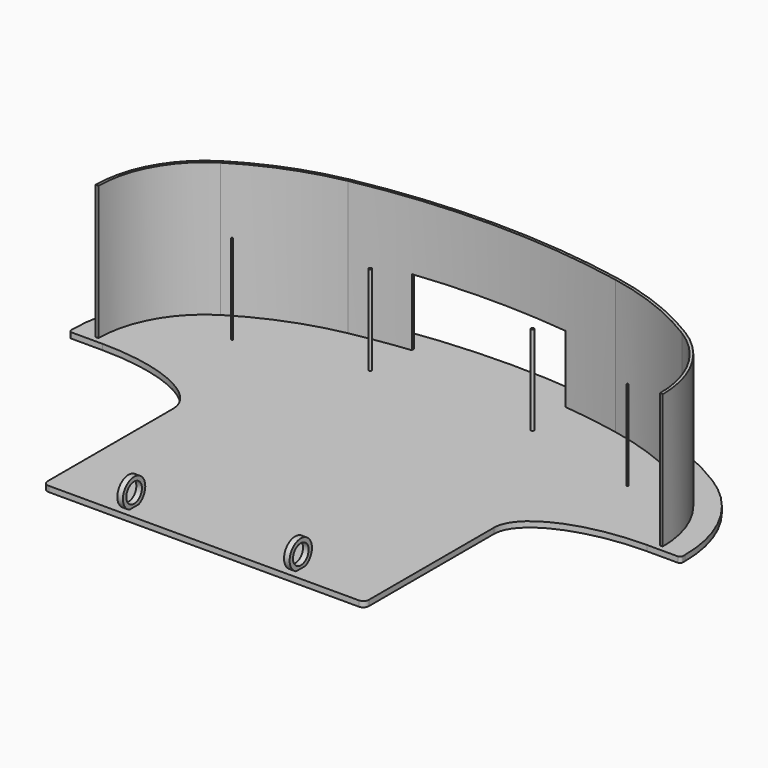
from build123d import *

# Parameters (mm, degrees)
F1_DEPTH  = 12.7
F3_R      = 31.75
F3_R_2    = 22.225
F4_DEPTH  = 12.7
F5_R      = 1.5875
F5_R_2    = 3.175
F6_DEPTH  = 203.2
F10_DEPTH = 304.8
F11_W     = 349.25
F11_H     = 152.4
F12_DEPTH = 876.3010001


# Not quite as in the source:
# - ends of sketch curves that miss each other by under 0.0002 mm in the source are joined
# - a feature of the source that left no trace in its solid (it failed there, or was rolled back) is left out
# - a pattern or mirror of a feature is missing from the dataset's text; its kind, count and spacing are read off the source's solid


with BuildPart() as f1:
    # F0 (on Top) → F1 (new body)
    with BuildSketch(Plane.XY):
        with BuildLine():
            Line((-599.0488908, 46.9398096), (-599.0488908, 40.5898096))
            ThreePointArc((-599.0488908, 40.5898096), (-597.1890188605, 36.0996815395), (-592.6988908, 34.2398096))
            Line((-592.6988908, 34.2398096), (-522.8488908, 34.2398096))
            add(Edge.make_bspline(
                [(-268.8488908, -83.2351904), (-268.8488908, 34.2397712098), (-522.8488908, 34.2398096)],
                knots=[0, 0, 0, 1.570796, 1.570796, 1.570796], degree=2, weights=[1, 0.7071068967, 1]))
            Line((-268.8488908, -83.2351904), (-268.8488908, -438.8351904))
            ThreePointArc((-268.8488908, -438.8351904), (-265.1291469211, -447.8154465211), (-256.1488908, -451.5351904))
            Line((-256.1488908, -451.5351904), (448.7011092, -451.5351904))
            ThreePointArc((448.7011092, -451.5351904), (457.6813653211, -447.8154465211), (461.4011092, -438.8351904))
            Line((461.4011092, -438.8351904), (461.4011092, -83.2351904))
            add(Edge.make_bspline(
                [(715.4011042177, 34.2398096), (461.4011872236, 34.2398072957), (461.4011092, -83.2351904)],
                knots=[4.712389, 4.712389, 4.712389, 6.283185, 6.283185, 6.283185], degree=2, weights=[1, 0.7071068967, 1]))
            Line((715.4011042177, 34.2398096), (785.2511092, 34.2398096))
            ThreePointArc((785.2511092, 34.2398096), (789.7412372605, 36.0996815395), (791.6011092, 40.5898096))
            Line((791.6011092, 40.5898096), (791.6011092, 46.9398096))
            ThreePointArc((791.6011092, 46.9398096), (753.9970119259, 191.9633164225), (650.6608007323, 300.4414852816))
            ThreePointArc((650.6608007323, 300.4414852816), (535.0314824748, 358.4359268507), (410.8101236244, 394.5267587894))
            ThreePointArc((410.8101236244, 394.5267587894), (96.2761092, 424.7648096), (-218.2579085609, 394.5267759822))
            ThreePointArc((-218.2579085609, 394.5267759822), (-342.4792640748, 358.4359268507), (-458.1085745053, 300.4414726845))
            ThreePointArc((-458.1085745053, 300.4414726845), (-561.4447935259, 191.9633164225), (-599.0488908, 46.9398096))
        make_face()
    extrude(amount=F1_DEPTH)

    # F3 (on offset) → F4 (join)
    with BuildSketch(Plane.YZ.offset(279.4)):
        with Locations((-420.6445217133, 41.4921417832)):
            Circle(F3_R)
        with Locations((-420.6445217133, 41.4921417832)):
            Circle(F3_R_2, mode=Mode.SUBTRACT)
    f4 = extrude(amount=F4_DEPTH)

    # F4_copies: F4 across plane
    add(f4.mirror(Plane(origin=(96.276109, 0, 0), x_dir=(0, 0, -1), z_dir=(-1, 0, 0))))

    # F5 (on face) → F6 (join)
    with BuildSketch(Plane.XY.offset(12.7)):
        with Locations((545.5359220505, 190.6074881554)):
            Circle(F5_R)
        with Locations((280.7082656561, 252.0138544033)):
            Circle(F5_R_2)
    f6 = extrude(amount=F6_DEPTH)

    # F6_copies: F6 across plane
    add(f6.mirror(Plane(origin=(96.276109, 0, 0), x_dir=(0, 0, -1), z_dir=(-1, 0, 0))))

    # F9 (on face) → F10 (join)
    with BuildSketch(Plane.XY.offset(12.7)):
        with BuildLine():
            Line((734.4511103495, 46.9398096), (740.8011092, 46.9398096))
            ThreePointArc((740.8011092, 46.9398096), (709.5977093343, 167.2784641974), (623.8506404715, 257.292263889))
            ThreePointArc((623.8506404715, 257.292263889), (516.4805587409, 311.1442444042), (401.1321540941, 344.6571597759))
            ThreePointArc((401.1321540941, 344.6571597759), (96.2761092, 373.9648096), (-208.5799387837, 344.6571770166))
            ThreePointArc((-208.5799387837, 344.6571770166), (-323.9283403409, 311.1442444042), (-431.2984143121, 257.2922512499))
            ThreePointArc((-431.2984143121, 257.2922512499), (-517.0454909343, 167.2784641974), (-548.2488908, 46.9398096))
            Line((-548.2488908, 46.9398096), (-541.8989002521, 46.9398096))
            ThreePointArc((-541.8989002521, 46.9398096), (-511.4955863715, 164.1928622622), (-427.9471570273, 251.8986192435))
            ThreePointArc((-427.9471570273, 251.8986192435), (-321.6094769175, 305.2327893075), (-207.3701905688, 338.4234653923))
            ThreePointArc((-207.3701905688, 338.4234653923), (96.2761092, 367.6148096), (399.9224109615, 338.4234771459))
            ThreePointArc((399.9224109615, 338.4234771459), (514.1616980249, 305.2327962096), (620.4993695539, 251.8986096209))
            ThreePointArc((620.4993695539, 251.8986096209), (704.047797515, 164.1928582278), (734.4511103495, 46.9398096))
        make_face()
    extrude(amount=F10_DEPTH)

    # F11 (on face) → F12 (cut, through all)
    with BuildSketch(Plane.XZ.offset(451.5351904)):
        with Locations((96.2761092, 88.9)):
            Rectangle(F11_W, F11_H)
    extrude(amount=-F12_DEPTH, mode=Mode.SUBTRACT)


solid = f1.part
